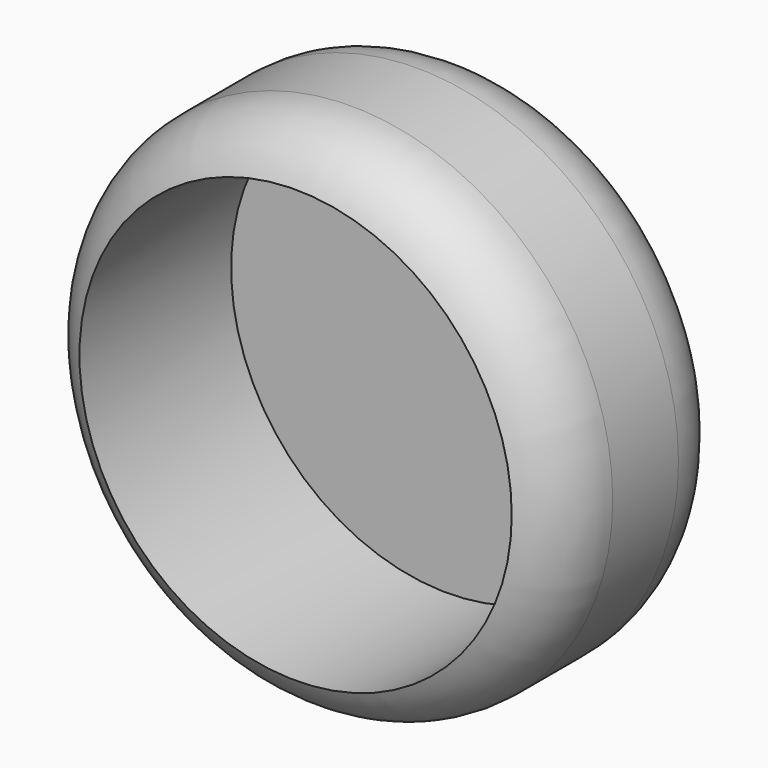
from build123d import *

# Parameters (mm, degrees)
F0_R     = 14.478
F1_DEPTH = 2.54
F0_R_2   = 17.5196905757
F2_DEPTH = 15.24


# Not quite as in the source:
# - a fillet or chamfer that OpenCascade refuses, or shapes differently, is made with other operations: its cross-section is extruded or revolved along the edge and cut away or added


with BuildPart() as f1:
    # F0 (on Front) → F1 (new body)
    with BuildSketch(Plane.XZ):
        Circle(F0_R)
    extrude(amount=F1_DEPTH)

    # F0 (on Front) → F2 (join)
    with BuildSketch(Plane.XZ):
        Circle(F0_R_2)
        Circle(F0_R, mode=Mode.SUBTRACT)
    extrude(amount=F2_DEPTH)

    # F3: fillet of radius 5.08 on 3 edges, made by hand

    # F3_s1 → F3_t2 (revolve, cut)
    with BuildSketch(Plane.XY):
        with BuildLine():
            ThreePointArc((12.4396905757, 0), (16.0317930242, -1.4878975516), (17.5196905757, -5.08))
            Line((17.5196905757, -5.08), (17.6212905757, -5.08))
            Line((17.6212905757, -5.08), (17.6212905757, 0.1016))
            Line((17.6212905757, 0.1016), (12.4396905757, 0.1016))
            Line((12.4396905757, 0.1016), (12.4396905757, 0))
        make_face()
    revolve(axis=Axis((0, 0, 0), (0, -1, 0)), mode=Mode.SUBTRACT)

    # F3_s3 → F3_t4 (revolve, cut)
    with BuildSketch(Plane.XY):
        with BuildLine():
            ThreePointArc((17.5196905757, -10.5868618448), (16.6918083937, -13.3664111001), (14.478, -15.24))
            Line((14.478, -15.24), (14.5187661885, -15.3330627631))
            ThreePointArc((14.5187661885, -15.3330627631), (15.9988452879, -15.3416), (17.5196905757, -15.3416))
            Line((17.5196905757, -15.3416), (17.6212905757, -15.24))
            Line((17.6212905757, -15.24), (17.6212905757, -10.5868618448))
            Line((17.6212905757, -10.5868618448), (17.5196905757, -10.5868618448))
        make_face()
    revolve(axis=Axis((0, -15.24, 0), (0, -1, 0)), mode=Mode.SUBTRACT)


solid = f1.part
